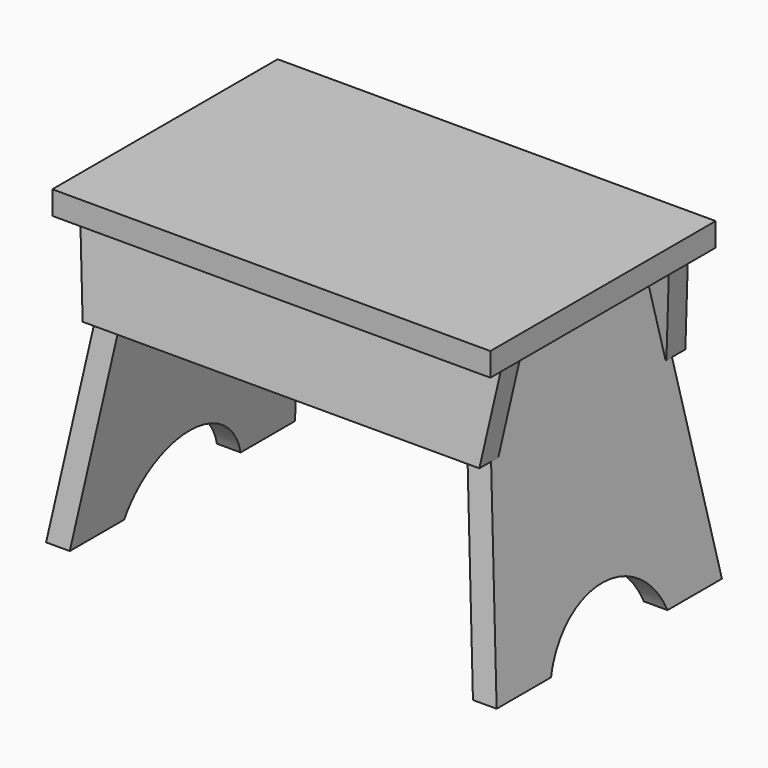
from build123d import *

# Parameters (mm, degrees)
F1_DEPTH      = 114.3
F2_DEPTH      = 114.3
F2_DEPTH_BACK = 114.3
F4_DEPTH      = 182.881
F4_DEPTH_BACK = 182.881
F6_DEPTH      = 177.8
F6_DEPTH_BACK = 177.8
F7_DEPTH      = 114.301
F7_DEPTH_BACK = 114.301
F8_DEPTH      = 177.8
F8_DEPTH_BACK = 177.8
F13_DEPTH     = 114.301
F14_DEPTH     = 114.301


# Not quite as in the source:
# - a feature names something its author has since deleted; it is built from what else it names


with BuildPart() as f1:
    # F0 (on Front) → F1 (new body, symmetric)
    with BuildSketch(Plane.XZ):
        Polygon((177.8, 9.525), (-177.8, 9.525), (-177.8, -9.525), (-171.45, -9.525), (-149.8599308867, -9.525), (-130.6227156302, -9.525), (130.6227156302, -9.525), (149.8599308867, -9.525), (171.45, -9.525), (177.8, -9.525), align=None)
    extrude(amount=F1_DEPTH, both=True)


with BuildPart() as f2:
    # F0 (on Front) → F2 (new body, two sides)
    with BuildSketch(Plane.XZ) as f2_sk:
        Polygon((-141.0489184441, -83.7112878215), (-160.2861337006, -83.7112878215), (-182.88, -244.475), (-163.6427847435, -244.475), align=None)
        Polygon((-130.6227156302, -9.525), (-149.8599308867, -9.525), (-160.2861337006, -83.7112878215), (-141.0489184441, -83.7112878215), align=None)
    extrude(amount=F2_DEPTH)
    extrude(f2_sk.sketch, amount=-F2_DEPTH_BACK)


with BuildPart() as f2b:
    # F0 (on Front) → F2, piece 2 (new body, two sides)
    with BuildSketch(Plane.XZ) as f2_2_sk:
        Polygon((182.88, -244.475), (160.2861337006, -83.7112878215), (141.0489184441, -83.7112878215), (163.6427847435, -244.475), align=None)
        Polygon((160.2861337006, -83.7112878215), (149.8599308867, -9.525), (130.6227156302, -9.525), (141.0489184441, -83.7112878215), align=None)
    extrude(amount=F2_DEPTH)
    extrude(f2_2_sk.sketch, amount=-F2_DEPTH_BACK)


with BuildPart() as f4_tool:
    # F3 (on Right) → F4 (new body, two sides)
    with BuildSketch(Plane.YZ) as f4_sk:
        Polygon((-114.3, -244.475), (-81.2799308867, -9.525), (-114.3000000004, -9.525), align=None)
        with BuildLine():
            Line((-59.0733587742, -244.475), (59.0733587742, -244.475))
            ThreePointArc((59.0733587742, -244.475), (0, -202.8182030655), (-59.0733587742, -244.475))
        make_face()
        Polygon((114.3, -244.475), (114.3, -9.525), (81.2799308867, -9.525), align=None)
    extrude(amount=-F4_DEPTH)
    extrude(f4_sk.sketch, amount=F4_DEPTH_BACK)


with BuildPart() as f2_1:
    add(f2.part)

    # F4: cut by f4_tool
    add(f4_tool.part, mode=Mode.SUBTRACT)


with BuildPart() as f2b_1:
    add(f2b.part)

    # F4: cut by f4_tool
    add(f4_tool.part, mode=Mode.SUBTRACT)


with BuildPart() as f6:
    # F5 (on Right) → F6 (new body, two sides)
    with BuildSketch(Plane.YZ) as f6_sk:
        Polygon((-91.7061337006, -83.7112878215), (-81.2799308867, -9.525), (-94.1047410577, -9.525), (-104.5309438716, -83.7112878215), align=None)
        Polygon((-74.8675258012, -9.525), (-81.2799308867, -9.525), (-91.7061337006, -83.7112878215), (-85.2937286151, -83.7112878215), align=None)
    extrude(amount=F6_DEPTH)
    extrude(f6_sk.sketch, amount=-F6_DEPTH_BACK)

    # F0 (on Front) → F7 (cut, two sides)
    with BuildSketch(Plane.XZ) as f7_sk:
        Polygon((-171.45, -9.525), (-177.8, -9.525), (-177.8, -83.7112878215), (-161.0237971861, -83.7112878215), align=None)
        Polygon((177.8, -83.7112878215), (177.8, -9.525), (171.45, -9.525), (161.0237971861, -83.7112878215), align=None)
    extrude(amount=-F7_DEPTH, mode=Mode.SUBTRACT)
    extrude(f7_sk.sketch, amount=F7_DEPTH_BACK, mode=Mode.SUBTRACT)

    # F10: cut F2
    add(f2_1.part, mode=Mode.SUBTRACT)

    # F11: cut F2b
    add(f2b_1.part, mode=Mode.SUBTRACT)


with BuildPart() as f8:
    # F5 (on Right) → F8 (new body, two sides)
    with BuildSketch(Plane.YZ) as f8_sk:
        Polygon((94.1047410577, -9.525), (81.2799308867, -9.525), (91.7061337006, -83.7112878215), (104.5309438716, -83.7112878215), align=None)
        Polygon((81.2799308867, -9.525), (74.8675258012, -9.525), (85.2937286151, -83.7112878215), (91.7061337006, -83.7112878215), align=None)
    extrude(amount=-F8_DEPTH)
    extrude(f8_sk.sketch, amount=F8_DEPTH_BACK)

    # F9: cut F2
    add(f2_1.part, mode=Mode.SUBTRACT)

    # F12: cut F2b
    add(f2b_1.part, mode=Mode.SUBTRACT)

    # F0 (on Front) → F13 (cut, through all)
    with BuildSketch(Plane.XZ):
        Polygon((177.8, -83.7112878215), (177.8, -9.525), (171.45, -9.525), (161.0237971861, -83.7112878215), align=None)
    extrude(amount=-F13_DEPTH, mode=Mode.SUBTRACT)

    # F0 (on Front) → F14 (cut, through all)
    with BuildSketch(Plane.XZ):
        Polygon((-171.45, -9.525), (-177.8, -9.525), (-177.8, -83.7112878215), (-161.0237971861, -83.7112878215), align=None)
    extrude(amount=-F14_DEPTH, mode=Mode.SUBTRACT)


solid = Compound([f1.part, f2_1.part, f2b_1.part, f6.part, f8.part])
